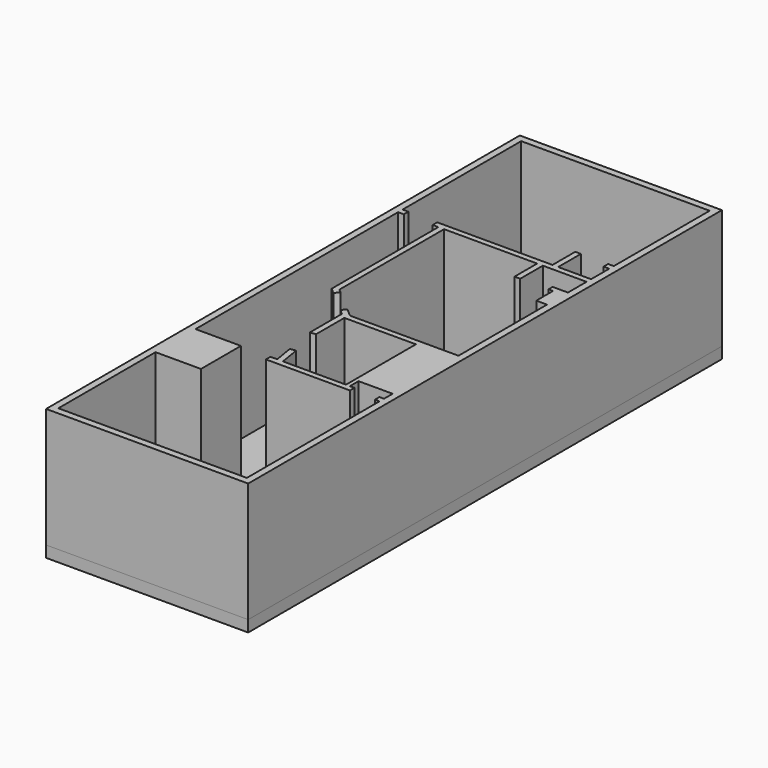
from build123d import *

# Parameters (mm, degrees)
F1_W     = 4521.2
F1_H     = 13246.1
F2_DEPTH = 254
F3_DEPTH = 2679.7


# Not quite as in the source:
# - a feature names something its author has since deleted; it is built from what else it names


with BuildPart() as f2:
    # F1 (on offset) → F2 (new body)
    with BuildSketch(Plane.XY.offset(2933.7)):
        with Locations((2108.2, 6470.65)):
            Rectangle(F1_W, F1_H)
        Polygon((4216.4, 0), (0, 0), (0, 2717.8), (1016, 2717.8), (1016, 3835.4), (0, 3835.4), (0, 9499.6), (127, 9499.6), (127, 9626.6), (0, 9626.6), (0, 12941.3), (4216.4, 12941.3), (4216.4, 10261.6), (4089.4, 10261.6), (4089.4, 10134.6), (4216.4, 10134.6), (4216.4, 9626.6), (3479.8, 9626.6), (3479.8, 10261.6), (3352.8, 10261.6), (3352.8, 9626.6), (774.7, 9626.6), (774.7, 9499.6), (901.7, 9499.6), (901.7, 6515.1), (1026.7483846603, 6407.2996683963), (1109.6717166631, 6503.4907335196), (1028.7, 6573.2939375395), (1028.7, 9499.6), (3111.5, 9499.6), (3111.5, 8864.6), (3238.5, 8864.6), (3238.5, 9499.6), (4216.4, 9499.6), (4216.4, 8978.9), (3873.5, 8978.9), (3873.5, 8864.6), (3975.1, 8864.6), (3975.1, 8394.7), (4216.4, 8394.7), (4216.4, 5918.2), (1788.6089675458, 5918.2), (1605.7940538549, 6075.7990635267), (1522.8707218521, 5979.6079984034), (1638.3, 5880.1), (1638.3, 4991.1), (1639.9617752246, 4980.9286603364), (1765.3, 5001.4061946153), (1765.3, 5791.2), (3365.5, 5791.2), (3365.5, 3835.4), (1955.8, 3835.4), (1879.9741919622, 4299.512135873), (1754.6359671868, 4279.034601594), (1827.1161924154, 3835.4), (1676.4, 3835.4), (1676.4, 3708.4), (3556, 3708.4), (3556, 3835.4), (3454.4, 3835.4), (3454.4, 4076.7), (4216.4, 4076.7), (4216.4, 3835.4), (4114.8, 3835.4), (4114.8, 3708.4), (4216.4, 3708.4), align=None, mode=Mode.SUBTRACT)
        Polygon((0, 2717.8), (0, 0), (4216.4, 0), (4216.4, 3708.4), (4114.8, 3708.4), (4114.8, 3835.4), (4216.4, 3835.4), (4216.4, 4076.7), (3454.4, 4076.7), (3454.4, 3835.4), (3556, 3835.4), (3556, 3708.4), (1676.4, 3708.4), (1676.4, 3835.4), (1827.1161924154, 3835.4), (1754.6359671868, 4279.034601594), (1879.9741919622, 4299.512135873), (1955.8, 3835.4), (3365.5, 3835.4), (3365.5, 5791.2), (1765.3, 5791.2), (1765.3, 5001.4061946153), (1639.9617752246, 4980.9286603364), (1638.3, 4991.1), (1638.3, 5880.1), (1522.8707218521, 5979.6079984034), (1605.7940538549, 6075.7990635267), (1788.6089675458, 5918.2), (4216.4, 5918.2), (4216.4, 8394.7), (3975.1, 8394.7), (3975.1, 8864.6), (3873.5, 8864.6), (3873.5, 8978.9), (4216.4, 8978.9), (4216.4, 9499.6), (3238.5, 9499.6), (3238.5, 8864.6), (3111.5, 8864.6), (3111.5, 9499.6), (1028.7, 9499.6), (1028.7, 6573.2939375395), (1109.6717166631, 6503.4907335196), (1026.7483846603, 6407.2996683963), (901.7, 6515.1), (901.7, 9499.6), (774.7, 9499.6), (774.7, 9626.6), (3352.8, 9626.6), (3352.8, 10261.6), (3479.8, 10261.6), (3479.8, 9626.6), (4216.4, 9626.6), (4216.4, 10134.6), (4089.4, 10134.6), (4089.4, 10261.6), (4216.4, 10261.6), (4216.4, 12941.3), (0, 12941.3), (0, 9626.6), (127, 9626.6), (127, 9499.6), (0, 9499.6), (0, 3835.4), (1016, 3835.4), (1016, 2717.8), align=None)
    extrude(amount=-F2_DEPTH)


with BuildPart() as f3:
    # F1 (on offset) → F3 (new body)
    with BuildSketch(Plane.XY.offset(2933.7)):
        with Locations((2108.2, 6470.65)):
            Rectangle(F1_W, F1_H)
        Polygon((4216.4, 0), (0, 0), (0, 2717.8), (1016, 2717.8), (1016, 3835.4), (0, 3835.4), (0, 9499.6), (127, 9499.6), (127, 9626.6), (0, 9626.6), (0, 12941.3), (4216.4, 12941.3), (4216.4, 10261.6), (4089.4, 10261.6), (4089.4, 10134.6), (4216.4, 10134.6), (4216.4, 9626.6), (3479.8, 9626.6), (3479.8, 10261.6), (3352.8, 10261.6), (3352.8, 9626.6), (774.7, 9626.6), (774.7, 9499.6), (901.7, 9499.6), (901.7, 6515.1), (1026.7483846603, 6407.2996683963), (1109.6717166631, 6503.4907335196), (1028.7, 6573.2939375395), (1028.7, 9499.6), (3111.5, 9499.6), (3111.5, 8864.6), (3238.5, 8864.6), (3238.5, 9499.6), (4216.4, 9499.6), (4216.4, 8978.9), (3873.5, 8978.9), (3873.5, 8864.6), (3975.1, 8864.6), (3975.1, 8394.7), (4216.4, 8394.7), (4216.4, 5918.2), (1788.6089675458, 5918.2), (1605.7940538549, 6075.7990635267), (1522.8707218521, 5979.6079984034), (1638.3, 5880.1), (1638.3, 4991.1), (1639.9617752246, 4980.9286603364), (1765.3, 5001.4061946153), (1765.3, 5791.2), (3365.5, 5791.2), (3365.5, 3835.4), (1955.8, 3835.4), (1879.9741919622, 4299.512135873), (1754.6359671868, 4279.034601594), (1827.1161924154, 3835.4), (1676.4, 3835.4), (1676.4, 3708.4), (3556, 3708.4), (3556, 3835.4), (3454.4, 3835.4), (3454.4, 4076.7), (4216.4, 4076.7), (4216.4, 3835.4), (4114.8, 3835.4), (4114.8, 3708.4), (4216.4, 3708.4), align=None, mode=Mode.SUBTRACT)
    extrude(amount=F3_DEPTH)


solid = Compound([f2.part, f3.part])
